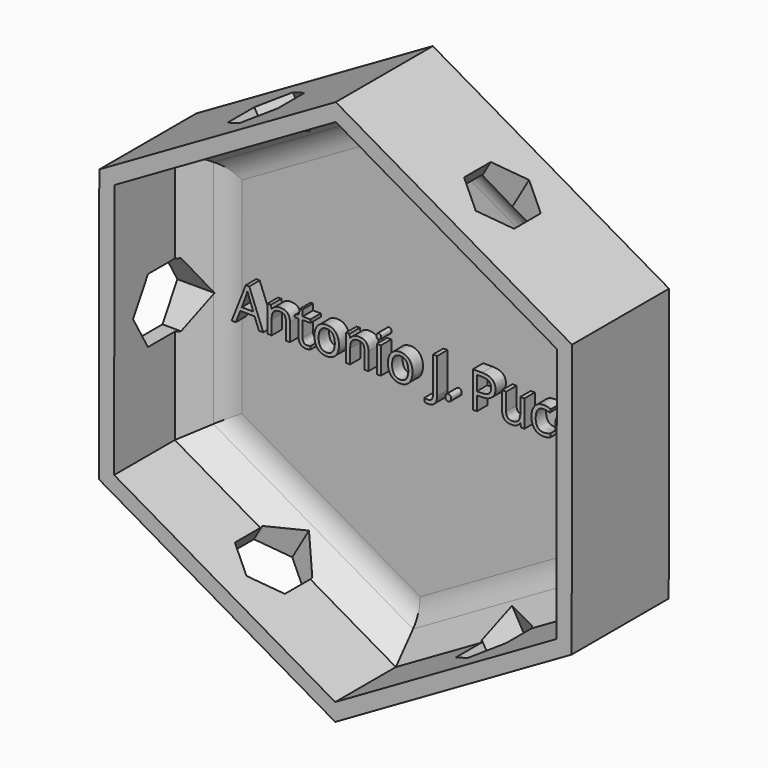
from build123d import *

# Parameters (mm, degrees)
F1_DEPTH      = 25.4
F2_T          = -2.54
F3_DEPTH      = 5.08
F4_SIZE       = 5.08
F5_R          = 5.08
F8_DEPTH      = 72.39
F9_DEPTH      = 92.202
F11_DEPTH     = 87.63
F12_TEXT_SIZE = 8.3721719707
F13_DEPTH     = 2.1844


# Not quite as in the source:
# - Text() gives the source's letters only with a copy of the font that has no kerning and outlines rounded to 1/6400 em; it was checked with that copy


with BuildPart() as f1:
    # F0 (on Front) → F1 (new body)
    with BuildSketch(Plane.XZ):
        Polygon((39.5686675606, -22.9049983078), (39.6206441885, 22.8149721475), (0.0519766279, 45.7199704553), (-39.5686675606, 22.9049983078), (-39.6206441885, -22.8149721475), (-0.0519766279, -45.7199704553), align=None)
    extrude(amount=F1_DEPTH)

    # F2
    f2_openings = [f1.faces().sort_by_distance(p)[0] for p in [
        (0, -25.4, 0),
    ]]
    offset(amount=F2_T, openings=f2_openings)

    # F3 (cut): a face of the model
    f3_faces = [f1.faces().sort_by_distance(p)[0] for p in [
        (19.1545486015, -25.4, -33.2639264176),
    ]]
    extrude(f3_faces, amount=-F3_DEPTH, mode=Mode.SUBTRACT)

    # F4
    f4_edges = [f1.edges().sort_by_distance(p)[0] for p in [
        (18.490847, -2.54, -32.111337),
        (37.054658, -2.54, -0.042125),
        (18.563811, -2.54, 32.069212),
        (-18.490847, -2.54, 32.111337),
        (-37.054658, -2.54, 0.042125),
        (-18.563811, -2.54, -32.069212),
    ]]
    chamfer(f4_edges, length=F4_SIZE)

    # F5
    f5_edges = [f1.edges().sort_by_distance(p)[0] for p in [
        (15.95585, -2.54, -27.709044),
        (-16.018811, -2.54, -27.672693),
        (31.974661, -2.54, -0.03635),
        (-31.974661, -2.54, 0.03635),
        (16.018811, -2.54, 27.672693),
        (-15.95585, -2.54, 27.709044),
    ]]
    fillet(f5_edges, radius=F5_R)

    # F7 (on face) → F8 (cut)
    with BuildSketch(Plane(origin=(-39.5946558745, 0, 0.0450130802), x_dir=(0, -1, 0), z_dir=(-0.9999993538, 0, 0.0011368466))):
        Polygon((13.2725168633, -5.3910373467), (16.3850337267, 0), (13.2725168633, 5.3910373467), (7.0474831367, 5.3910373467), (3.9349662733, 0), (7.0474831367, -5.3910373467), align=None)
    extrude(amount=-F8_DEPTH, mode=Mode.SUBTRACT)

    # F6 (on face) → F9 (cut)
    with BuildSketch(Plane(origin=(-19.8363104082, 0, -34.2674713014), x_dir=(0.8654564208, 0, -0.500984215), z_dir=(-0.500984215, 0, -0.8654564208))):
        Polygon((4.8385803115, 12.9535556453), (0, 15.7471112907), (-4.8385803115, 12.9535556453), (-4.8385803115, 7.3664443547), (0, 4.5728887093), (4.8385803115, 7.3664443547), align=None)
    extrude(amount=-F9_DEPTH, mode=Mode.SUBTRACT)

    # F10 (on face) → F11 (cut)
    with BuildSketch(Plane(origin=(-19.7583454663, 0, 34.3124843815), x_dir=(0.8665932675, 0, 0.4990151388), z_dir=(-0.4990151388, 0, 0.8665932675))):
        Polygon((-4.8572535342, -12.9643366355), (0, -15.7686732709), (4.8572535342, -12.9643366355), (4.8572535342, -7.3556633645), (0, -4.5513267291), (-4.8572535342, -7.3556633645), align=None)
    extrude(amount=-F11_DEPTH, mode=Mode.SUBTRACT)

    # F12 (on face) → F13 (join)
    with BuildSketch(Plane.XZ.offset(2.54)):
        with Locations((-29.8665794862, -2.5830153572)):
            Text('Antonio J. Pucci', F12_TEXT_SIZE, font='Open Sans', text_align=(TextAlign.LEFT, TextAlign.BOTTOM))
    extrude(amount=F13_DEPTH)


solid = f1.part
